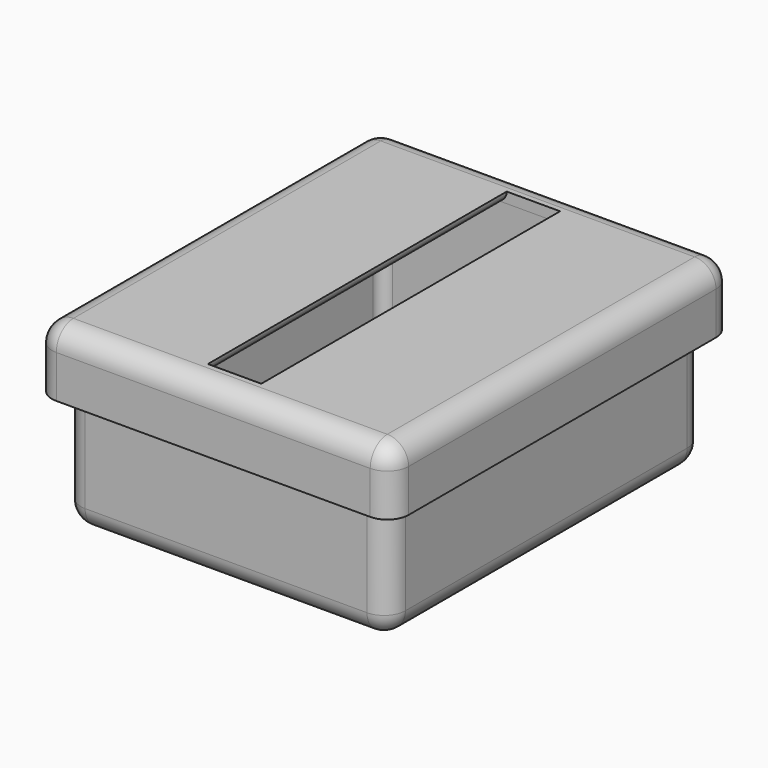
from build123d import *

# Parameters (mm, degrees)
F3_W          = 60.8333333333
F3_H          = 74
F4_DEPTH      = 32
F5_T          = -2
F6_R          = 2
F7_R          = 4
F8_W          = 66.8333333333
F8_H          = 80
F9_DEPTH      = 2
F9_DEPTH_BACK = 10
F10_T         = -2
F11_W         = 10
F11_H         = 70
F12_DEPTH     = 2.001
F14_DEPTH     = 17.5
F15_R         = 1.99999
F16_R         = 4


# Not quite as in the source:
# - a fillet or chamfer is up to 0.001 mm smaller than in the source, because OpenCascade refuses the exact size


with BuildPart() as f4:
    # F3 (on Top) → F4 (new body, through all)
    with BuildSketch(Plane.XY):
        Rectangle(F3_W, F3_H)
    extrude(amount=F4_DEPTH)

    # F5
    f5_openings = [f4.faces().sort_by_distance(p)[0] for p in [
        (0, 0, 32),
    ]]
    offset(amount=F5_T, openings=f5_openings)

    # F6
    f6_edges = [f4.edges().sort_by_distance(p)[0] for p in [
        (0, -35, 2),
        (28.416667, 0, 2),
        (0, 35, 2),
        (-28.416667, 0, 2),
        (28.416667, -35, 17),
        (28.416667, 35, 17),
        (-28.416667, 35, 17),
        (-28.416667, -35, 17),
    ]]
    fillet(f6_edges, radius=F6_R)

    # F7
    f7_edges = [f4.edges().sort_by_distance(p)[0] for p in [
        (0, -37, 0),
        (30.416667, 0, 0),
        (0, 37, 0),
        (-30.416667, 0, 0),
        (30.416667, -37, 16),
        (30.416667, 37, 16),
        (-30.416667, -37, 16),
        (-30.416667, 37, 16),
    ]]
    fillet(f7_edges, radius=F7_R)


with BuildPart() as f9:
    # F8 (on offset) → F9 (new body, two sides)
    with BuildSketch(Plane.XY.offset(32)) as f9_sk:
        Rectangle(F8_W, F8_H)
    extrude(amount=F9_DEPTH)
    extrude(f9_sk.sketch, amount=-F9_DEPTH_BACK)

    # F10
    f10_openings = [f9.faces().sort_by_distance(p)[0] for p in [
        (0, 0, 22),
    ]]
    offset(amount=F10_T, openings=f10_openings)

    # F11 (on offset) → F12 (cut, through all)
    with BuildSketch(Plane.XY.offset(32)):
        Rectangle(F11_W, F11_H)
    extrude(amount=F12_DEPTH, mode=Mode.SUBTRACT)

    # F13 (on Front) → F14 (join, symmetric)
    with BuildSketch(Plane.XZ):
        Polygon((-30.4166666667, 26.7320508076), (-31.4166666667, 27.7320508076), (-31.4166666667, 22), (-30.4166666667, 23.7320508076), align=None)
        Polygon((31.4166666667, 22), (31.4166666667, 27.7320508076), (30.4166666667, 26.7320508076), (30.4166666667, 23.7320508076), align=None)
    extrude(amount=F14_DEPTH, both=True)

    # F15 (radius 2 in the source; OpenCascade refuses exactly that, so slightly less here)
    f15_edges = [f9.edges().sort_by_distance(p)[0] for p in [
        (0, -38, 32),
        (-31.416667, 0, 32),
        (0, 38, 32),
        (31.416667, 0, 32),
        (5, 0, 32),
        (-5, 0, 32),
        (-31.416667, -38, 27),
        (31.416667, -38, 27),
        (31.416667, 38, 27),
        (-31.416667, 38, 27),
    ]]
    fillet(f15_edges, radius=F15_R)

    # F16
    f16_edges = [f9.edges().sort_by_distance(p)[0] for p in [
        (33.416667, 0, 34),
        (-33.416667, 0, 34),
        (0, 40, 34),
        (0, -40, 34),
        (33.416667, -40, 28),
        (33.416667, 40, 28),
        (-33.416667, 40, 28),
        (-33.416667, -40, 28),
    ]]
    fillet(f16_edges, radius=F16_R)


solid = Compound([f4.part, f9.part])
